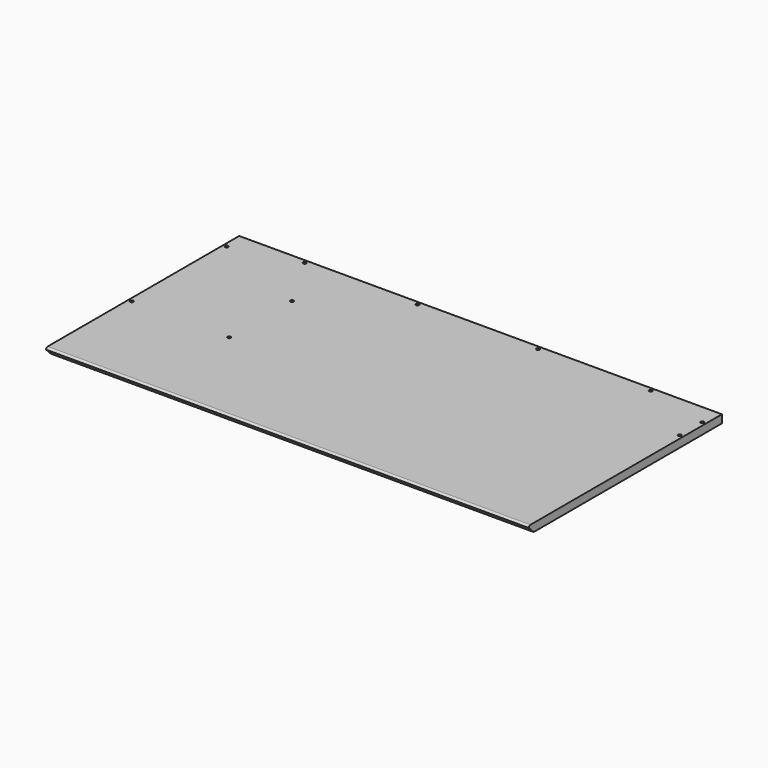
from build123d import *

# Parameters (mm, degrees)
F0_W           = 1200
F0_H           = 600
F1_DEPTH       = 20
F2_R           = 5
F3_SIZE        = 14.99999
F6_D           = 8
F6_DEPTH       = 10
F6_TIP         = 2.4034424761
F6_ON_F5_D     = 8
F6_ON_F5_DEPTH = 10
F6_ON_F5_TIP   = 2.4034424761


# Not quite as in the source:
# - a fillet or chamfer is up to 0.001 mm smaller than in the source, because OpenCascade refuses the exact size


with BuildPart() as f1:
    # F0 (on Top) → F1 (new body)
    with BuildSketch(Plane.XY):
        with Locations((600, -300)):
            Rectangle(F0_W, F0_H)
    extrude(amount=F1_DEPTH)

    # F2
    f2_edges = [f1.edges().sort_by_distance(p)[0] for p in [
        (600, -600, 20),
    ]]
    fillet(f2_edges, radius=F2_R)

    # F3 (size 15 in the source; OpenCascade refuses exactly that, so slightly less here)
    f3_edges = [f1.edges().sort_by_distance(p)[0] for p in [
        (600, -600, 0),
    ]]
    chamfer(f3_edges, length=F3_SIZE)

    # F6
    with Locations(Plane.XY.offset(20)):
        with Locations((1030, -9), (750, -9), (450, -9), (170, -9), (9, -50), (9, -345), (251, -150), (251, -345), (1191, -120), (1191, -50)):
            Hole(F6_D / 2, depth=F6_DEPTH)
            with Locations((0, 0, -(F6_DEPTH + F6_TIP / 2))):  # 118° drill point
                Cone(0, F6_D / 2, F6_TIP, mode=Mode.SUBTRACT)

    # F6 on F5
    with Locations(Plane(origin=(0, 0, 0), x_dir=(1, 0, 0), z_dir=(0, 0, -1))):
        with Locations((189, 482.5), (189, 102.5), (1011, 102.5), (1011, 482.5)):
            Hole(F6_ON_F5_D / 2, depth=F6_ON_F5_DEPTH)
            with Locations((0, 0, -(F6_ON_F5_DEPTH + F6_ON_F5_TIP / 2))):  # 118° drill point
                Cone(0, F6_ON_F5_D / 2, F6_ON_F5_TIP, mode=Mode.SUBTRACT)


solid = f1.part
